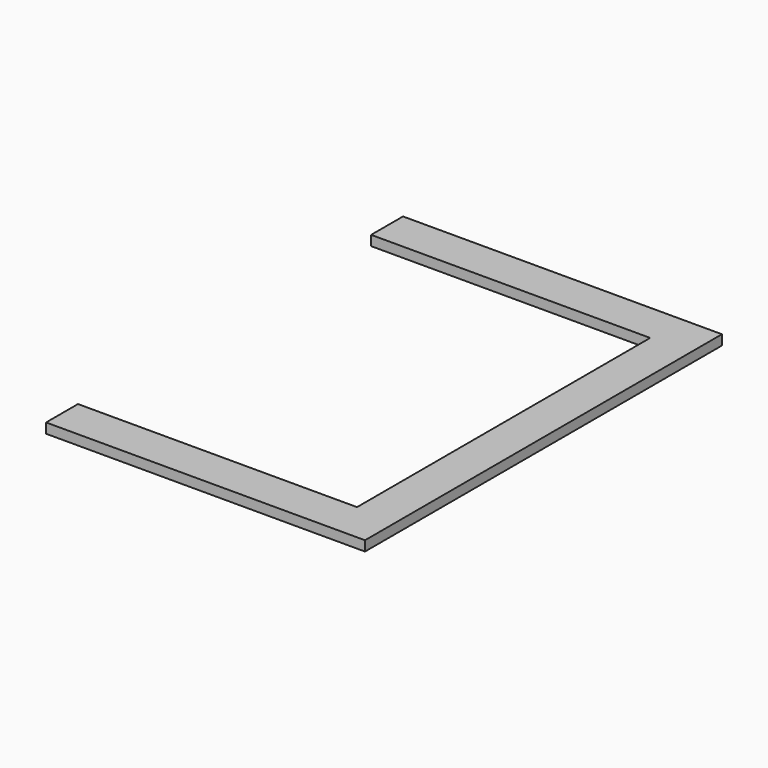
from build123d import *

# Parameters (mm, degrees)
F0_W     = 12.7
F0_H     = 233.4768
F1_DEPTH = 6.35


# Not quite as in the source:
# - a feature names something its author has since deleted; it is built from what else it names


with BuildPart() as f1:
    # F0 (on Top) → F1 (new body)
    with BuildSketch(Plane.XY):
        Polygon((88.9, -116.7384), (76.2, -116.7384), (-76.2, -116.7384), (-101.6, -116.7384), (-101.6, -142.1384), (101.6, -142.1384), (101.6, -116.7384), align=None)
        Polygon((-76.2, 116.7384), (76.2, 116.7384), (88.9, 116.7384), (101.6, 116.7384), (101.6, 142.1384), (-101.6, 142.1384), (-101.6, 116.7384), align=None)
        with Locations((95.25, 0)):
            Rectangle(F0_W, F0_H)
        with Locations((82.55, 0)):
            Rectangle(F0_W, F0_H)
    extrude(amount=F1_DEPTH)


solid = f1.part
